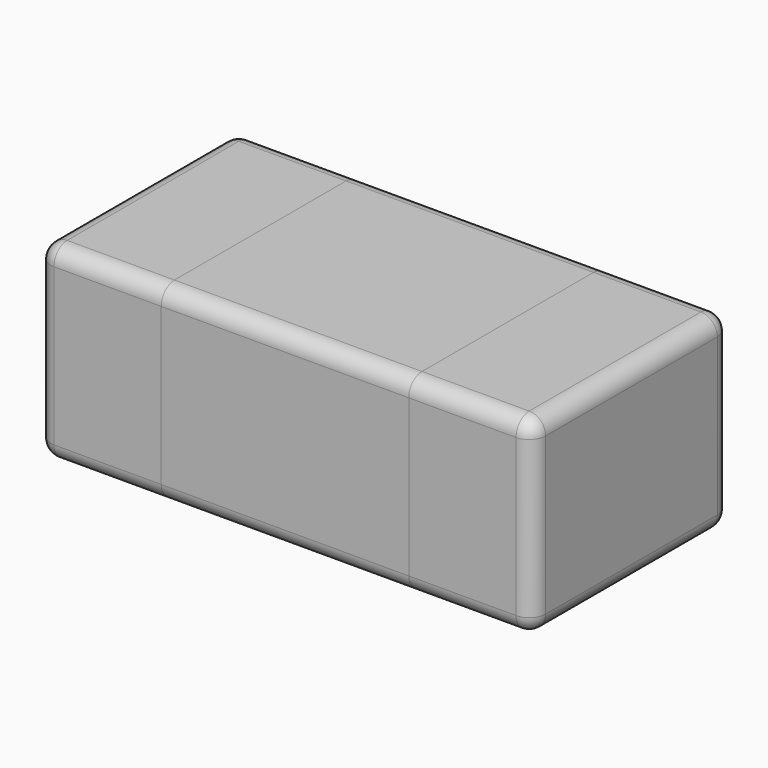
from build123d import *

# Parameters (mm, degrees)
F2_W     = 0.3
F2_H     = 0.3
F3_DEPTH = 0.21
F2_W_2   = 0.15
F4_DEPTH = 0.23
F5_DEPTH = 0.23
F6_DEPTH = 0.02
F7_R     = 0.01999
F7_2_R   = 0.01999
F7_3_R   = 0.01999
F7_4_R   = 0.01999


# Not quite as in the source:
# - a fillet or chamfer is up to 0.001 mm smaller than in the source, because OpenCascade refuses the exact size


with BuildPart() as f3:
    # F2 (on Top) → F3 (new body)
    with BuildSketch(Plane.XY):
        Rectangle(F2_W, F2_H)
    extrude(amount=F3_DEPTH)


with BuildPart() as f4:
    # F2 (on Top) → F4 (new body)
    with BuildSketch(Plane.XY):
        with Locations((-0.225, 0)):
            Rectangle(F2_W_2, F2_H)
    extrude(amount=F4_DEPTH)

    # F7 (radius 0.02 in the source; OpenCascade refuses exactly that, so slightly less here)
    f7_edges = [f4.edges().sort_by_distance(p)[0] for p in [
        (-0.225, -0.15, 0.23),
        (-0.3, 0.15, 0.115),
        (-0.3, -0.15, 0.115),
        (-0.3, 0, 0),
        (-0.3, 0, 0.23),
        (-0.225, 0.15, 0.23),
        (-0.225, 0.15, 0),
        (-0.225, -0.15, 0),
    ]]
    fillet(f7_edges, radius=F7_R)


with BuildPart() as f5:
    # F2 (on Top) → F5 (new body)
    with BuildSketch(Plane.XY):
        with Locations((0.225, 0)):
            Rectangle(F2_W_2, F2_H)
    extrude(amount=F5_DEPTH)

    # F7#2 (radius 0.02 in the source; OpenCascade refuses exactly that, so slightly less here)
    f7_2_edges = [f5.edges().sort_by_distance(p)[0] for p in [
        (0.225, -0.15, 0.23),
        (0.3, -0.15, 0.115),
        (0.3, 0.15, 0.115),
        (0.3, 0, 0),
        (0.3, 0, 0.23),
        (0.225, 0.15, 0.23),
        (0.225, 0.15, 0),
        (0.225, -0.15, 0),
    ]]
    fillet(f7_2_edges, radius=F7_2_R)


with BuildPart() as f6:
    # F6 (new): a face of the model
    f6_faces = [f3.part.faces().sort_by_distance(p)[0] for p in [
        (0, 0, 0.21),
    ]]
    extrude(f6_faces, amount=F6_DEPTH)

    # F7#4 (radius 0.02 in the source; OpenCascade refuses exactly that, so slightly less here)
    f7_4_edges = [f6.edges().sort_by_distance(p)[0] for p in [
        (0, -0.15, 0.23),
        (0, 0.15, 0.23),
    ]]
    fillet(f7_4_edges, radius=F7_4_R)


with BuildPart() as f3_1:
    add(f3.part)

    # F7#3 (radius 0.02 in the source; OpenCascade refuses exactly that, so slightly less here)
    f7_3_edges = [f3_1.edges().sort_by_distance(p)[0] for p in [
        (0, 0.15, 0),
        (0, -0.15, 0),
    ]]
    fillet(f7_3_edges, radius=F7_3_R)


solid = Compound([f4.part, f5.part, f6.part, f3_1.part])
